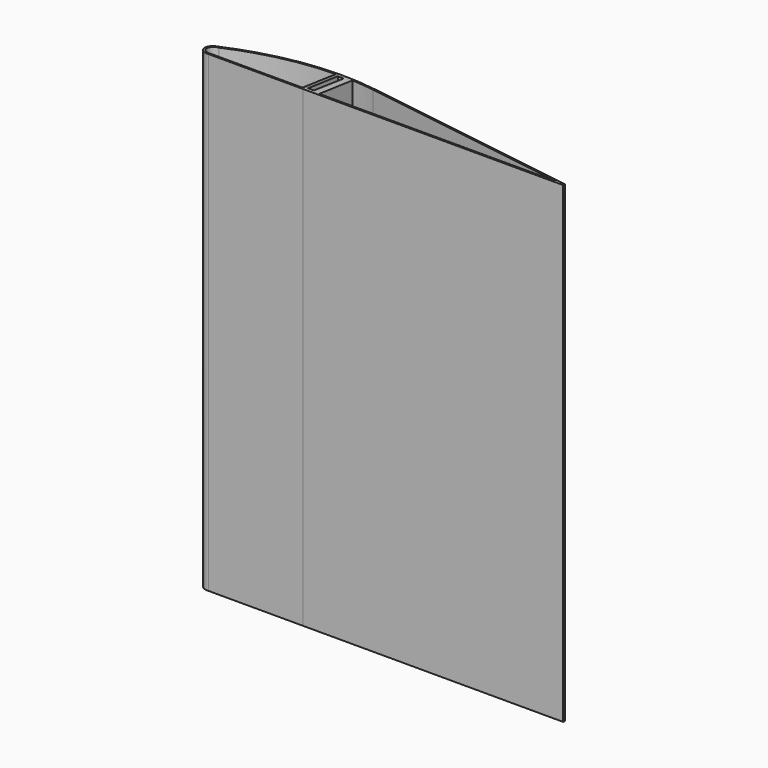
from build123d import *

# Parameters (mm, degrees)
F1_DEPTH     = 200
F3_DEPTH     = 200
F4_T         = -0.8
F4_2_T       = -0.8
F5_W         = 2.5
F5_H         = 1
F6_DEPTH     = 20
F7_T4_DEPTH  = 5.5
F7_T9_DEPTH  = 30.5
F7_T14_ANGLE = 37.7423343373
F7_T20_ANGLE = 37.7423343373
F8_W         = 155.1876314091
F8_H         = 22.3366669118
F9_ANGLE     = 7


# Not quite as in the source:
# - a fillet or chamfer that OpenCascade refuses, or shapes differently, is made with other operations: its cross-section is extruded or revolved along the edge and cut away or added


with BuildPart() as f1:
    # F0 (on Top) → F1 (new body)
    with BuildSketch(Plane.XY):
        with BuildLine():
            Line((94.1401966023, -3), (94.1696608117, -2.0004341641))
            Line((94.1696608117, -2.0004341641), (0, 15))
            ThreePointArc((0, 15), (-7.9879059152, 16.0504323354), (-16.0396361483, 16.3327251865))
            Line((-16.0396361483, 16.3327251865), (-16.0396361483, -3))
            Line((-16.0396361483, -3), (94.1401966023, -3))
        make_face()
    extrude(amount=F1_DEPTH)

    # F4
    f4_openings = [f1.faces().sort_by_distance(p)[0] for p in [
        (22.614044, 3.891358, 200),
    ]]
    offset(amount=F4_T, openings=f4_openings)

    # F5 (on face) → F6 (join)
    with BuildSketch(Plane.XY.offset(200)):
        Polygon((-12.7396361483, -1.2), (-12.7396361483, -2.2), (-9.7396361483, -2.2), (-9.7396361483, 15.5391672506), (-12.7396361483, 15.5391672506), (-12.7396361483, 14.5391672506), align=None)
        with Locations((-13.9896361483, -1.7)):
            Rectangle(F5_W, F5_H)
        with Locations((-13.9896361483, 15.0391672506)):
            Rectangle(F5_W, F5_H)
    extrude(amount=-F6_DEPTH)

    # F7: fillet of radius 10 on 2 edges, made by hand


with BuildPart() as f3:
    # F2 (on face) → F3 (new body)
    with BuildSketch(Plane.XY.offset(200)):
        with BuildLine():
            Line((-16.0396361483, -3), (-16.0396361483, 16.3327251865))
            ThreePointArc((-16.0396361483, 16.3327251865), (-37.5222437907, 13.2612199418), (-57.5066562048, 4.8019152395))
            ThreePointArc((-57.5066562048, 4.8019152395), (-60.2806962129, 0.1415930949), (-55.8598033977, -3))
            Line((-55.8598033977, -3), (-16.0396361483, -3))
        make_face()
    extrude(amount=-F3_DEPTH)

    # F4#2
    f4_2_openings = [f3.faces().sort_by_distance(p)[0] for p in [
        (-34.83961, 5.023506, 200),
    ]]
    offset(amount=F4_2_T, openings=f4_2_openings, kind=Kind.INTERSECTION)


with BuildPart() as f7_tool2:
    # F7_s3 → F7_t4 (new body)
    with BuildSketch(Plane.YZ.offset(-15.2396361483)):
        with BuildLine():
            ThreePointArc((-2.2, 170), (0.7289321881, 177.0710678119), (7.8, 180))
            Line((7.8, 180), (-2.2, 180))
            Line((-2.2, 180), (-2.2, 170))
        make_face()
    extrude(amount=F7_T4_DEPTH)

    split(bisect_by=Plane.XZ.offset(1.2), keep=Keep.TOP)


with BuildPart() as f1_1:
    add(f1.part)

    # F7_t1: union F7_tool2
    add(f7_tool2.part)


with BuildPart() as f7_tool7:
    # F7_s8 → F7_t9 (new body)
    with BuildSketch(Plane.YZ.offset(-40.2396361483)):
        with BuildLine():
            ThreePointArc((-2.2, 170), (0.7289321881, 177.0710678119), (7.8, 180))
            Line((7.8, 180), (-2.2, 180))
            Line((-2.2, 180), (-2.2, 170))
        make_face()
    extrude(amount=F7_T9_DEPTH)

    split(bisect_by=Plane.YZ.offset(-12.7396361483), keep=Keep.TOP)


with BuildPart() as f1_2:
    add(f1_1.part)

    # F7_t6: union F7_tool7
    add(f7_tool7.part)


with BuildPart() as f7_tool12:
    # F7_s13 → F7_t14 (revolve)
    with BuildSketch(Plane(origin=(-32.6433997569, -9.9682739464, 0), x_dir=(0, 0, 1), z_dir=(-0.9564014883, -0.2920551201, 0))):
        with BuildLine():
            ThreePointArc((170, 22.8682565899), (177.0710678119, 19.9393244018), (180, 12.8682565899))
            Line((180, 12.8682565899), (180, 22.8682565899))
            Line((180, 22.8682565899), (170, 22.8682565899))
        make_face()
    revolve(axis=Axis((-14.9610707823, -67.8731164952, 180), (0, 0, -1)), revolution_arc=F7_T14_ANGLE)

    split(bisect_by=Plane.YZ.offset(-12.7396361483), keep=Keep.TOP)

    split(bisect_by=Plane.YZ.offset(-9.7396361483), keep=Keep.BOTTOM)


with BuildPart() as f1_3:
    add(f1_2.part)

    # F7_t11: union F7_tool12
    add(f7_tool12.part)


with BuildPart() as f7_tool18:
    # F7_s19 → F7_t20 (revolve)
    with BuildSketch(Plane(origin=(-32.6433997569, -9.9682739464, 0), x_dir=(0, 0, 1), z_dir=(-0.9564014883, -0.2920551201, 0))):
        with BuildLine():
            ThreePointArc((170, 22.8682565899), (177.0710678119, 19.9393244018), (180, 12.8682565899))
            Line((180, 12.8682565899), (180, 22.8682565899))
            Line((180, 22.8682565899), (170, 22.8682565899))
        make_face()
    revolve(axis=Axis((-14.9610707823, -67.8731164952, 180), (0, 0, -1)), revolution_arc=F7_T20_ANGLE)

    split(bisect_by=Plane.YZ.offset(-15.2396361483), keep=Keep.TOP)

    split(bisect_by=Plane.XZ.offset(-14.5391672506), keep=Keep.BOTTOM)

    split(bisect_by=Plane.XZ.offset(-15.5391672506), keep=Keep.TOP)

    split(bisect_by=Plane.YZ.offset(-9.7396361483), keep=Keep.BOTTOM)


with BuildPart() as f1_4:
    add(f1_3.part)

    # F7_t17: union F7_tool18
    add(f7_tool18.part)


with BuildPart() as f9_tool:
    # F8 (on face) → F9 (revolve)
    with BuildSketch(Plane.XY.offset(200)):
        with Locations((16.5463808977, 8.1683334559)):
            Rectangle(F8_W, F8_H)
    revolve(axis=Axis((16.5463808977, -3, 200), (-1, 0, 0)), revolution_arc=F9_ANGLE)


with BuildPart() as f1_5:
    add(f1_4.part)

    # F9: cut by f9_tool
    add(f9_tool.part, mode=Mode.SUBTRACT)


with BuildPart() as f3_1:
    add(f3.part)

    # F9: cut by f9_tool
    add(f9_tool.part, mode=Mode.SUBTRACT)


solid = Compound([f1_5.part, f3_1.part])
